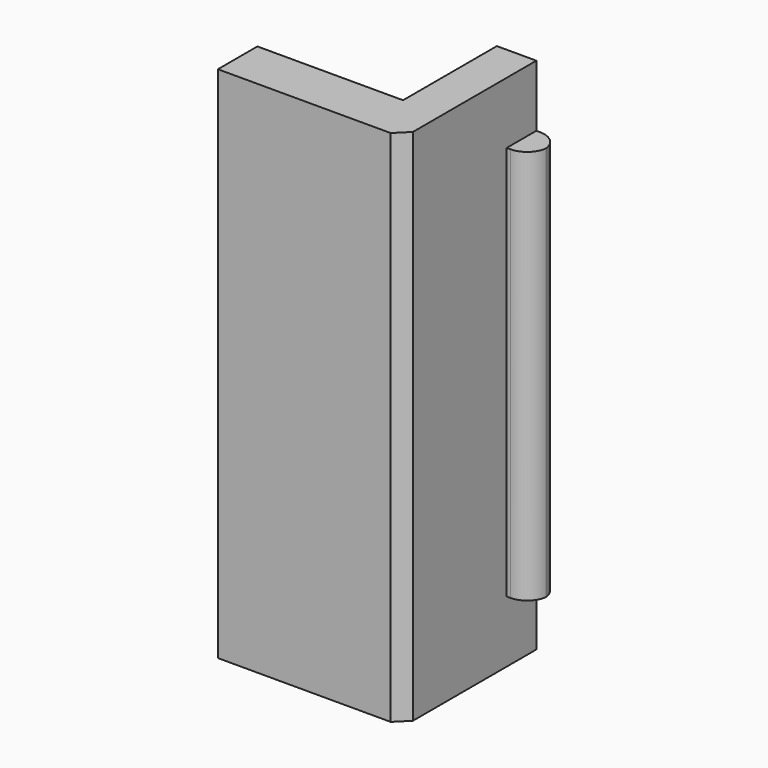
from build123d import *

# Parameters (mm, degrees)
F1_DEPTH    = 21
F2_START    = 2.5
F0_W        = 1
F0_H        = 1.5
F2_DEPTH    = 16
F3_SIZE     = 0.5
F4_T1_DEPTH = 20.25


# Not quite as in the source:
# - a fillet or chamfer that OpenCascade refuses, or shapes differently, is made with other operations: its cross-section is extruded or revolved along the edge and cut away or added


with BuildPart() as f1:
    # F0 (on Top) → F1 (new body)
    with BuildSketch(Plane.XY):
        Polygon((0, 2), (0, 0), (7.5, 0), (7.5, 5.25), (7.5, 6.75), (5.9, 6.75), (5.9, 2), align=None)
    extrude(amount=F1_DEPTH)

    # F0 (on Top) → F2 (join)
    with BuildSketch(Plane.XY.offset(F2_START)):
        with Locations((8, 6)):
            Rectangle(F0_W, F0_H)
    extrude(amount=F2_DEPTH)

    # F3
    f3_edges = [f1.edges().sort_by_distance(p)[0] for p in [
        (7.5, 0, 10.5),
    ]]
    chamfer(f3_edges, length=F3_SIZE)

    # F4: fillet of radius 0.85 on 2 edges, made by hand

    # F4_s2 → F4_t1 (cut)
    with BuildSketch(Plane.XY.offset(0.375)):
        with BuildLine():
            ThreePointArc((7.65, 6.75), (8.251040764, 6.501040764), (8.5, 5.9))
            Line((8.5, 5.9), (8.5, 6.75))
            Line((8.5, 6.75), (7.65, 6.75))
        make_face()
        with BuildLine():
            ThreePointArc((7.65, 5.25), (8.251040764, 5.498959236), (8.5, 6.1))
            Line((8.5, 6.1), (8.5, 5.25))
            Line((8.5, 5.25), (7.65, 5.25))
        make_face()
    extrude(amount=F4_T1_DEPTH, mode=Mode.SUBTRACT)


solid = f1.part
